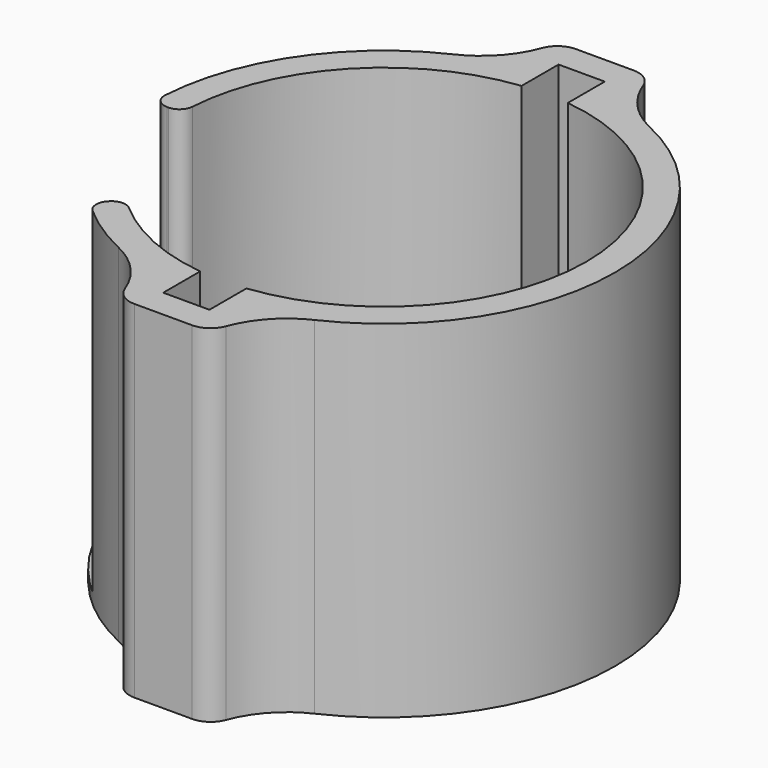
from build123d import *

# Parameters (mm, degrees)
F1_DEPTH    = 0.5999988
F2_DEPTH    = 19.05
F3_R        = 1.27
F4_R        = 5.08
F5_T1_DEPTH = 20.4776308939
F5_T3_DEPTH = 20.2938151504


# Not quite as in the source:
# - a fillet or chamfer that OpenCascade refuses, or shapes differently, is made with other operations: its cross-section is extruded or revolved along the edge and cut away or added


with BuildPart() as f1:
    # F0 (on Top) → F1 (new body)
    with BuildSketch(Plane.XY):
        with BuildLine():
            Line((-1.27, 13.5796900432), (-1.27, 11.0396900432))
            ThreePointArc((-1.27, 11.0396900432), (-8.2945925533, 7.3950923338), (-11.1125, 0))
            ThreePointArc((-11.1125, 0), (-10.266611305, -4.2525696422), (-7.8577241059, -7.8577241059))
            ThreePointArc((-7.8577241059, -7.8577241059), (-4.8332249736, -10.0063775966), (-1.27, -11.0396900432))
            Line((-1.27, -11.0396900432), (-1.27, -13.5796900432))
            Line((-1.27, -13.5796900432), (0, -13.5796900432))
            Line((0, -13.5796900432), (1.27, -13.5796900432))
            Line((1.27, -13.5796900432), (1.27, -11.0396900432))
            ThreePointArc((1.27, -11.0396900432), (11.1125, 0), (1.27, 11.0396900432))
            Line((1.27, 11.0396900432), (1.27, 13.5796900432))
            Line((1.27, 13.5796900432), (0, 13.5796900432))
            Line((0, 13.5796900432), (-1.27, 13.5796900432))
        make_face()
        with BuildLine():
            ThreePointArc((-7.8577241059, -7.8577241059), (-10.266611305, -4.2525696422), (-11.1125, 0))
            Line((-11.1125, 0), (-12.7, 0))
            ThreePointArc((-12.7, 0), (-11.7332700629, -4.860079591), (-8.9802561211, -8.9802561211))
            Line((-8.9802561211, -8.9802561211), (-7.8577241059, -7.8577241059))
        make_face()
    extrude(amount=F1_DEPTH)

    # F0 (on Top) → F2 (join)
    with BuildSketch(Plane.XY):
        with BuildLine():
            ThreePointArc((-11.1125, 0), (-8.2945925533, 7.3950923338), (-1.27, 11.0396900432))
            Line((-1.27, 11.0396900432), (-1.27, 13.5796900432))
            Line((-1.27, 13.5796900432), (0, 13.5796900432))
            Line((0, 13.5796900432), (1.27, 13.5796900432))
            Line((1.27, 13.5796900432), (1.27, 11.0396900432))
            ThreePointArc((1.27, 11.0396900432), (11.1125, 0), (1.27, -11.0396900432))
            Line((1.27, -11.0396900432), (1.27, -13.5796900432))
            Line((1.27, -13.5796900432), (0, -13.5796900432))
            Line((0, -13.5796900432), (-1.27, -13.5796900432))
            Line((-1.27, -13.5796900432), (-1.27, -11.0396900432))
            ThreePointArc((-1.27, -11.0396900432), (-4.8332249736, -10.0063775966), (-7.8577241059, -7.8577241059))
            Line((-7.8577241059, -7.8577241059), (-8.9802561211, -8.9802561211))
            ThreePointArc((-8.9802561211, -8.9802561211), (-6.1573611633, -11.1075156315), (-2.8575, -12.3743562964))
            Line((-2.8575, -12.3743562964), (-2.8575, -15.1671900432))
            Line((-2.8575, -15.1671900432), (0, -15.1671900432))
            Line((0, -15.1671900432), (2.8575, -15.1671900432))
            Line((2.8575, -15.1671900432), (2.8575, -12.3743562964))
            ThreePointArc((2.8575, -12.3743562964), (12.7, 0), (2.8575, 12.3743562964))
            Line((2.8575, 12.3743562964), (2.8575, 15.1671900432))
            Line((2.8575, 15.1671900432), (0, 15.1671900432))
            Line((0, 15.1671900432), (-2.8575, 15.1671900432))
            Line((-2.8575, 15.1671900432), (-2.8575, 12.3743562964))
            ThreePointArc((-2.8575, 12.3743562964), (-9.93932216, 7.9056862447), (-12.7, 0))
            Line((-12.7, 0), (-11.1125, 0))
        make_face()
    extrude(amount=F2_DEPTH)

    # F3
    f3_edges = [f1.edges().sort_by_distance(p)[0] for p in [
        (2.8575, -15.16719, 9.525),
        (-2.8575, -15.16719, 9.525),
        (-2.8575, 15.16719, 9.525),
        (2.8575, 15.16719, 9.525),
    ]]
    fillet(f3_edges, radius=F3_R)

    # F4
    f4_edges = [f1.edges().sort_by_distance(p)[0] for p in [
        (2.8575, 12.374356, 9.525),
        (-2.8575, 12.374356, 9.525),
        (-2.8575, -12.374356, 9.525),
        (2.8575, -12.374356, 9.525),
    ]]
    fillet(f4_edges, radius=F4_R)

    # F5: fillet of radius 0.762 on 4 edges, made by hand

    # F5_s2 → F5_t1 (cut)
    with BuildSketch(Plane.XY.offset(0.5999988)):
        with BuildLine():
            ThreePointArc((-12.6741021595, 0.8106382979), (-12.4694016476, 0.2406643993), (-11.91365603, 0))
            Line((-11.91365603, 0), (-12.7, 0))
            ThreePointArc((-12.7, 0), (-12.6935238887, 0.4055259388), (-12.6741021595, 0.8106382979))
        make_face()
        with BuildLine():
            ThreePointArc((-8.3887357449, -9.53515142), (-8.6470230336, -8.9873738911), (-8.4242269675, -8.4242269675))
            Line((-8.4242269675, -8.4242269675), (-8.9802561211, -8.9802561211))
            ThreePointArc((-8.9802561211, -8.9802561211), (-8.6889266776, -9.2624269601), (-8.3887357449, -9.53515142))
        make_face()
    extrude(amount=F5_T1_DEPTH, mode=Mode.SUBTRACT)

    # F5_s4 → F5_t3 (cut)
    with BuildSketch(Plane.XY.offset(0.5999988)):
        with BuildLine():
            ThreePointArc((-11.8500255801, 0), (-11.3287850299, 0.2061652325), (-11.0895961312, 0.7131016043))
            ThreePointArc((-11.0895961312, 0.7131016043), (-11.1067725568, 0.3567346651), (-11.1125, 0))
            Line((-11.1125, 0), (-11.8500255801, 0))
        make_face()
        with BuildLine():
            ThreePointArc((-8.379233445, -8.379233445), (-7.8648798833, -8.1564415512), (-7.3372896449, -8.345767605))
            ThreePointArc((-7.3372896449, -8.345767605), (-7.6014246912, -8.1059236928), (-7.8577241059, -7.8577241059))
            Line((-7.8577241059, -7.8577241059), (-8.379233445, -8.379233445))
        make_face()
    extrude(amount=F5_T3_DEPTH, mode=Mode.SUBTRACT)


solid = f1.part
